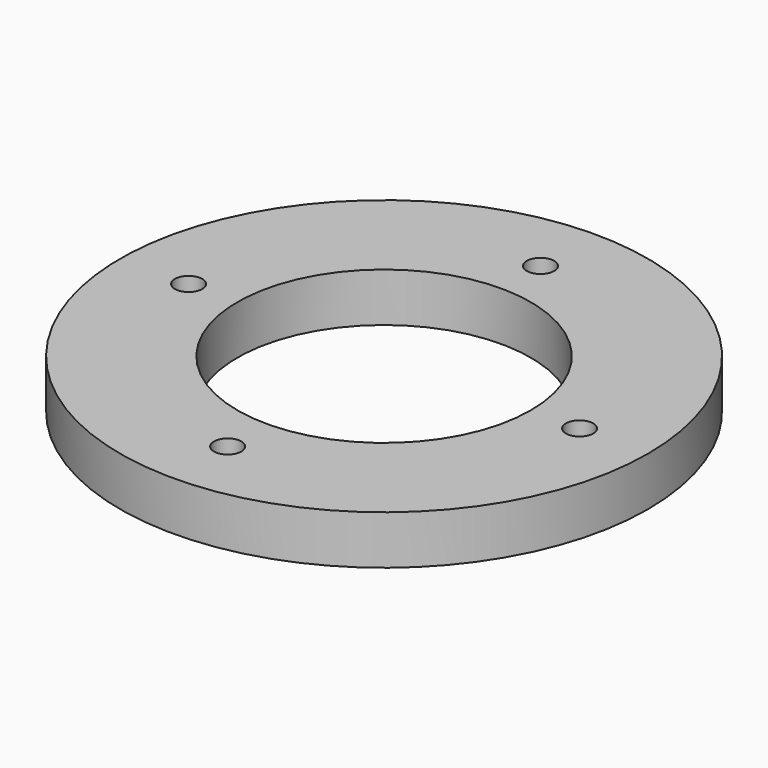
from build123d import *

# Parameters (mm, degrees)
F0_R     = 34.29
F0_R_2   = 1.778
F0_R_3   = 19.05
F1_DEPTH = 6.35


# Not quite as in the source:
# - a length typed as a fraction of an inch, garbled in the dataset ("3 / 203.2 mm" for 3/8 in), is restored


with BuildPart() as f1:
    # F0 (on Top) → F1 (new body)
    with BuildSketch(Plane.XY):
        Circle(F0_R)
        with Locations((0, -25.4)):
            Circle(F0_R_2, mode=Mode.SUBTRACT)
        with Locations((-25.4, 0)):
            Circle(F0_R_2, mode=Mode.SUBTRACT)
        Circle(F0_R_3, mode=Mode.SUBTRACT)
        with Locations((25.4, 0)):
            Circle(F0_R_2, mode=Mode.SUBTRACT)
        with Locations((0, 25.4)):
            Circle(F0_R_2, mode=Mode.SUBTRACT)
    extrude(amount=F1_DEPTH)


solid = f1.part
